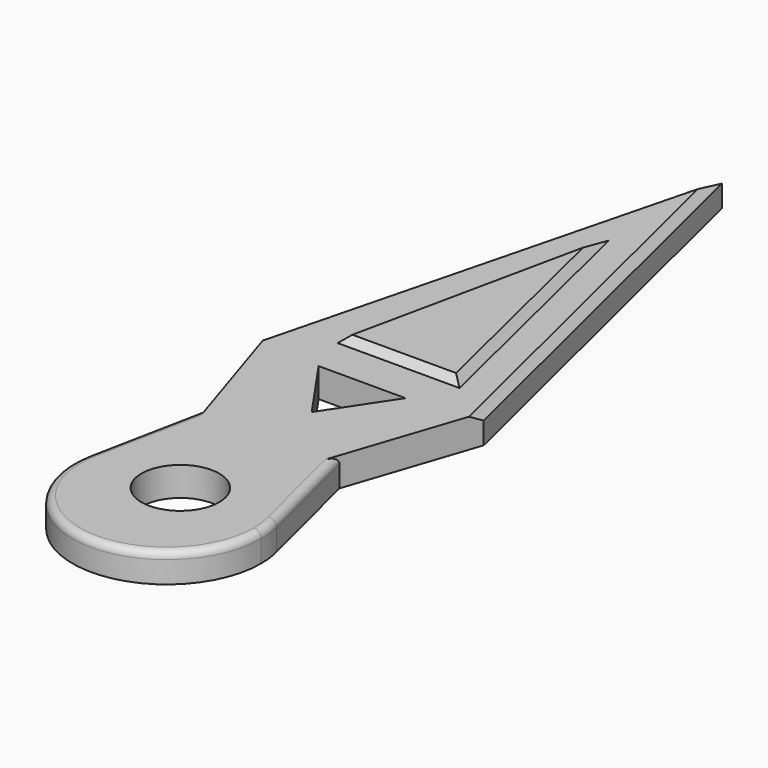
from build123d import *

# Parameters (mm, degrees)
F1_DEPTH = 4
F2_R     = 5.3437499794
F3_DEPTH = 25.4
F5_DEPTH = 25.4
F7_DEPTH = 1
F8_SIZE  = 0.99999
F9_SIZE  = 0.99999
F10_SIZE = 1
F11_R    = 1


# Not quite as in the source:
# - a fillet or chamfer is up to 0.001 mm smaller than in the source, because OpenCascade refuses the exact size


with BuildPart() as f1:
    # F0 (on Top) → F1 (new body)
    with BuildSketch(Plane.XY):
        Polygon((0, 76.4742046595), (-15.0523874909, 17.476933077), (14.446250163, 17.476933077), align=None)
        with BuildLine():
            Line((14.446250163, 17.476933077), (-15.0523874909, 17.476933077))
            Line((-15.0523874909, 17.476933077), (-9.4487972359, 0))
            Line((-9.4487972359, 0), (-12.7043901229, -16.3636804159))
            ThreePointArc((-12.7043901229, -16.3636804159), (-0.3230678893, -5.9418952878), (12.5625447422, -15.7333064535))
            Line((12.5625447422, -15.7333064535), (8.6075438617, 0))
            Line((8.6075438617, 0), (14.446250163, 17.476933077))
        make_face()
        with BuildLine():
            ThreePointArc((12.5625447422, -15.7333064535), (-0.3230678893, -5.9418952878), (-12.7043901229, -16.3636804159))
            ThreePointArc((-12.7043901229, -16.3636804159), (-1.2699015357, -31.782233325), (12.9533829787, -18.891248852))
            ThreePointArc((12.9533829787, -18.891248852), (12.8553020934, -17.3002307252), (12.5625447422, -15.7333064535))
        make_face()
    extrude(amount=F1_DEPTH)

    # F2 (on face) → F3 (cut)
    with BuildSketch(Plane.XY.offset(4)):
        with Locations((0, -16.5616404265)):
            Circle(F2_R)
    extrude(amount=-F3_DEPTH, mode=Mode.SUBTRACT)

    # F4 (on face) → F5 (cut)
    with BuildSketch(Plane.XY.offset(4)):
        Polygon((-6.0996017419, 14.8122329265), (0, 6.0074422508), (5.8425283059, 14.8122329265), align=None)
    extrude(amount=-F5_DEPTH, mode=Mode.SUBTRACT)

    # F6 (on face) → F7 (join)
    with BuildSketch(Plane.XY.offset(4)):
        Polygon((0, 57.0488348603), (-7.8442301601, 20.2657673508), (8.901366964, 20.2657673508), align=None)
    extrude(amount=F7_DEPTH)

    # F8 (size 1 in the source; OpenCascade refuses exactly that, so slightly less here)
    f8_edges = [f1.edges().sort_by_distance(p)[0] for p in [
        (-3.922115, 38.657301, 5),
        (4.450683, 38.657301, 5),
    ]]
    chamfer(f8_edges, length=F8_SIZE)

    # F9 (size 1 in the source; OpenCascade refuses exactly that, so slightly less here)
    f9_edges = [f1.edges().sort_by_distance(p)[0] for p in [
        (0.525379, 20.265767, 5),
    ]]
    chamfer(f9_edges, length=F9_SIZE)

    # F10
    f10_edges = [f1.edges().sort_by_distance(p)[0] for p in [
        (-7.526194, 46.975569, 4),
        (7.223125, 46.975569, 4),
    ]]
    chamfer(f10_edges, length=F10_SIZE)

    # F11
    f11_edges = [f1.edges().sort_by_distance(p)[0] for p in [
        (0.323068, -31.840602, 4),
    ]]
    fillet(f11_edges, radius=F11_R)


solid = f1.part
